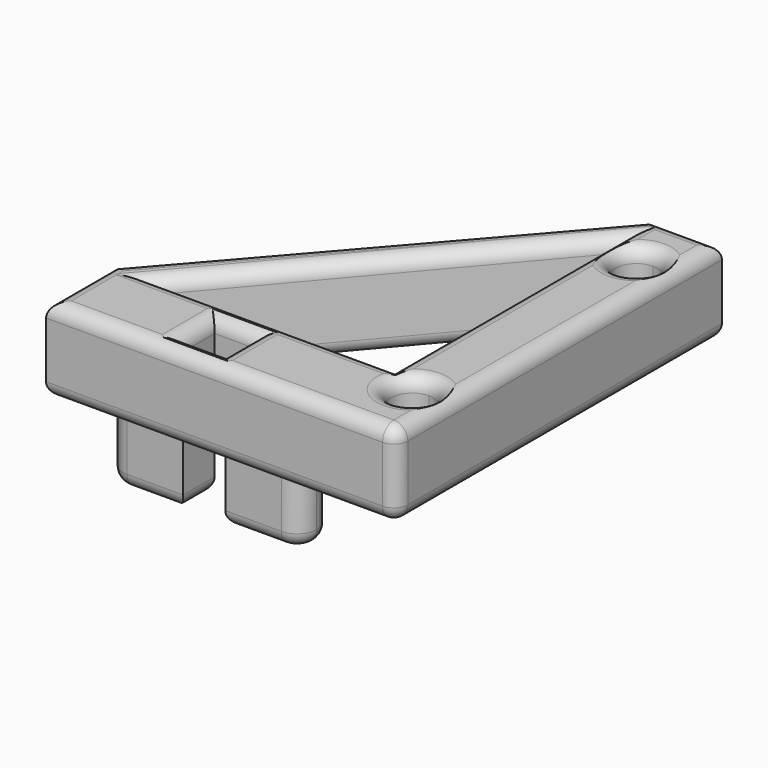
from build123d import *

# Parameters (mm, degrees)
F1_DEPTH      = 6
F2_DEPTH      = 6
F3_T1_DEPTH   = 35.4795013083
F3_T3_DEPTH   = 11
F3_T5_DEPTH   = 30
F3_T7_DEPTH   = 34
F3_T9_DEPTH   = 10
F3_T11_DEPTH  = 3
F3_T13_DEPTH  = 2.8
F3_T18_DEPTH  = 31.2488094968
F3_T24_DEPTH  = 22.5
F3_T29_DEPTH  = 19.5
F3_T39_DEPTH  = 5.5
F3_T43_DEPTH  = 5.3
F3_T50_DEPTH  = 5.5
F3_T54_DEPTH  = 5.3
F3_T61_DEPTH  = 5.3
F3_T65_DEPTH  = 5.5
F3_T72_DEPTH  = 5.5
F3_T76_DEPTH  = 5.3
F3_T83_DEPTH  = 31.2488094968
F3_T87_DEPTH  = 19.5
F3_T94_DEPTH  = 31.2488094968
F3_T98_DEPTH  = 22.5
F3_T105_DEPTH = 25
F3_T109_DEPTH = 22
F4_T1_DEPTH   = 35.4795013083
F4_T3_DEPTH   = 11
F4_T5_DEPTH   = 26.5
F4_T7_DEPTH   = 30.5
F4_T9_DEPTH   = 10
F4_T11_DEPTH  = 3
F4_T13_DEPTH  = 2.8
F4_T15_DEPTH  = 4
F4_S19_W      = 1
F4_S19_H      = 1
F4_T20_DEPTH  = 1
F4_S25_W      = 1
F4_S25_H      = 1
F4_T26_DEPTH  = 1
F4_T32_DEPTH  = 31.2488094968
F4_T38_DEPTH  = 22.5
F4_T43_DEPTH  = 19.5
F4_T53_DEPTH  = 5.5
F4_T57_DEPTH  = 5.3
F4_T64_DEPTH  = 5.5
F4_T68_DEPTH  = 5.3
F4_T75_DEPTH  = 5.5
F4_T79_DEPTH  = 5.3
F4_T86_DEPTH  = 5.3
F4_T90_DEPTH  = 5.5
F4_T97_DEPTH  = 31.2488094968
F4_T101_DEPTH = 19.5
F4_T108_DEPTH = 22.5
F4_T112_DEPTH = 31.2488094968
F4_T119_DEPTH = 25
F4_T123_DEPTH = 22
F5_DEPTH      = 5
F6_R          = 1


# Not quite as in the source:
# - a fillet or chamfer that OpenCascade refuses, or shapes differently, is made with other operations: its cross-section is extruded or revolved along the edge and cut away or added


with BuildPart() as f1:
    # F0 (on Top) → F1 (new body)
    with BuildSketch(Plane.XY):
        Polygon((0, 29), (-20, 6), (-17, 6), (0, 26), align=None)
        with BuildLine():
            Line((0, 3), (0, 0))
            Line((0, 0), (2.5, 0))
            Line((2.5, 0), (2.5, 3))
            ThreePointArc((2.5, 3), (1, 4.5), (2.5, 6))
            Line((2.5, 6), (2.5, 23))
            ThreePointArc((2.5, 23), (1, 24.5), (2.5, 26))
            Line((2.5, 26), (2.5, 29))
            Line((2.5, 29), (0, 29))
            Line((0, 29), (0, 26))
            Line((0, 26), (0, 6))
            Line((0, 6), (0, 3))
        make_face()
        with BuildLine():
            Line((2.5, 3), (2.5, 0))
            Line((2.5, 0), (5, 0))
            Line((5, 0), (5, 15))
            Line((5, 15), (5, 29))
            Line((5, 29), (2.5, 29))
            Line((2.5, 29), (2.5, 26))
            ThreePointArc((2.5, 26), (3.5606601718, 25.5606601718), (4, 24.5))
            ThreePointArc((4, 24.5), (3.5606601718, 23.4393398282), (2.5, 23))
            Line((2.5, 23), (2.5, 6))
            ThreePointArc((2.5, 6), (3.5606601718, 5.5606601718), (4, 4.5))
            ThreePointArc((4, 4.5), (3.5606601718, 3.4393398282), (2.5, 3))
        make_face()
        with BuildLine():
            Line((-3.1, 3), (0, 3))
            Line((0, 3), (0, 6))
            Line((0, 6), (-17, 6))
            Line((-17, 6), (-20, 6))
            Line((-20, 6), (-20, 3))
            Line((-20, 3), (-16.9, 3))
            ThreePointArc((-16.9, 3), (-16.4899494937, 3.9899494937), (-15.5, 4.4))
            Line((-15.5, 4.4), (-11.5, 4.4))
            Line((-11.5, 4.4), (-10, 4.4))
            Line((-10, 4.4), (-8.5, 4.4))
            Line((-8.5, 4.4), (-4.5, 4.4))
            ThreePointArc((-4.5, 4.4), (-3.5100505063, 3.9899494937), (-3.1, 3))
        make_face()
        with BuildLine():
            Line((-20, 0), (0, 0))
            Line((0, 0), (0, 3))
            Line((0, 3), (-3.1, 3))
            ThreePointArc((-3.1, 3), (-3.5100505063, 2.0100505063), (-4.5, 1.6))
            Line((-4.5, 1.6), (-8.5, 1.6))
            Line((-8.5, 1.6), (-10, 1.6))
            Line((-10, 1.6), (-11.5, 1.6))
            Line((-11.5, 1.6), (-15.5, 1.6))
            ThreePointArc((-15.5, 1.6), (-16.4899494937, 2.0100505063), (-16.9, 3))
            Line((-16.9, 3), (-20, 3))
            Line((-20, 3), (-20, 0))
        make_face()
    extrude(amount=F1_DEPTH)

    # F0 (on Top) → F2 (join)
    with BuildSketch(Plane.XY):
        with BuildLine():
            Line((-14.1, 3), (-16.9, 3))
            ThreePointArc((-16.9, 3), (-16.4899494937, 2.0100505063), (-15.5, 1.6))
            ThreePointArc((-15.5, 1.6), (-14.5100505063, 2.0100505063), (-14.1, 3))
        make_face()
        with BuildLine():
            ThreePointArc((-4.5, 1.6), (-5.4899494937, 2.0100505063), (-5.9, 3))
            Line((-5.9, 3), (-8.5, 3))
            Line((-8.5, 3), (-8.5, 1.6))
            Line((-8.5, 1.6), (-4.5, 1.6))
        make_face()
        with BuildLine():
            Line((-11.5, 3), (-14.1, 3))
            ThreePointArc((-14.1, 3), (-14.5100505063, 2.0100505063), (-15.5, 1.6))
            Line((-15.5, 1.6), (-11.5, 1.6))
            Line((-11.5, 1.6), (-11.5, 3))
        make_face()
        with BuildLine():
            ThreePointArc((-15.5, 4.4), (-14.5100505063, 3.9899494937), (-14.1, 3))
            Line((-14.1, 3), (-11.5, 3))
            Line((-11.5, 3), (-11.5, 4.4))
            Line((-11.5, 4.4), (-15.5, 4.4))
        make_face()
        with BuildLine():
            Line((-8.5, 3), (-5.9, 3))
            ThreePointArc((-5.9, 3), (-5.4899494937, 3.9899494937), (-4.5, 4.4))
            Line((-4.5, 4.4), (-8.5, 4.4))
            Line((-8.5, 4.4), (-8.5, 3))
        make_face()
        with BuildLine():
            Line((-5.9, 3), (-3.1, 3))
            ThreePointArc((-3.1, 3), (-3.5100505063, 3.9899494937), (-4.5, 4.4))
            ThreePointArc((-4.5, 4.4), (-5.4899494937, 3.9899494937), (-5.9, 3))
        make_face()
        with BuildLine():
            ThreePointArc((-4.5, 1.6), (-3.5100505063, 2.0100505063), (-3.1, 3))
            Line((-3.1, 3), (-5.9, 3))
            ThreePointArc((-5.9, 3), (-5.4899494937, 2.0100505063), (-4.5, 1.6))
        make_face()
        with BuildLine():
            ThreePointArc((-15.5, 4.4), (-16.4899494937, 3.9899494937), (-16.9, 3))
            Line((-16.9, 3), (-14.1, 3))
            ThreePointArc((-14.1, 3), (-14.5100505063, 3.9899494937), (-15.5, 4.4))
        make_face()
    extrude(amount=F2_DEPTH)

    # F3: fillet of radius 1 on 14 edges, made by hand

    # F3_s2 → F3_t1 (cut)
    with BuildSketch(Plane(origin=(15.9999731598, 18.3999691337, 0), x_dir=(0, 0, 1), z_dir=(-0.6561787149, -0.7546055222, 0))):
        with BuildLine():
            ThreePointArc((5, 19.0291827328), (5.7071067812, 18.736289514), (6, 18.0291827328))
            Line((6, 18.0291827328), (6, 19.0291827328))
            Line((6, 19.0291827328), (5, 19.0291827328))
        make_face()
    extrude(amount=F3_T1_DEPTH, mode=Mode.SUBTRACT)

    # F3_s4 → F3_t3 (cut)
    with BuildSketch(Plane.XZ.offset(-8.5)):
        with BuildLine():
            ThreePointArc((-20, 5), (-19.7071067812, 5.7071067812), (-19, 6))
            Line((-19, 6), (-20, 6))
            Line((-20, 6), (-20, 5))
        make_face()
    extrude(amount=F3_T3_DEPTH, mode=Mode.SUBTRACT)

    # F3_s6 → F3_t5 (cut)
    with BuildSketch(Plane.YZ.offset(-22.5)):
        with BuildLine():
            ThreePointArc((1, 6), (0.2928932188, 5.7071067812), (0, 5))
            Line((0, 5), (0, 6))
            Line((0, 6), (1, 6))
        make_face()
    extrude(amount=F3_T5_DEPTH, mode=Mode.SUBTRACT)

    # F3_s8 → F3_t7 (cut)
    with BuildSketch(Plane.XZ.offset(-31.5)):
        with BuildLine():
            ThreePointArc((4, 6), (4.7071067812, 5.7071067812), (5, 5))
            Line((5, 5), (5, 6))
            Line((5, 6), (4, 6))
        make_face()
    extrude(amount=F3_T7_DEPTH, mode=Mode.SUBTRACT)

    # F3_s10 → F3_t9 (cut)
    with BuildSketch(Plane.YZ.offset(-2.5)):
        with BuildLine():
            ThreePointArc((29, 5), (28.7071067812, 5.7071067812), (28, 6))
            Line((28, 6), (29, 6))
            Line((29, 6), (29, 5))
        make_face()
    extrude(amount=F3_T9_DEPTH, mode=Mode.SUBTRACT)

    # F3_s12 → F3_t11 (cut)
    with BuildSketch(Plane.YZ.offset(-11.5)):
        with BuildLine():
            ThreePointArc((5.4, 6), (4.6928932188, 5.7071067812), (4.4, 5))
            Line((4.4, 5), (4.4, 6))
            Line((4.4, 6), (5.4, 6))
        make_face()
        with BuildLine():
            ThreePointArc((0.6, 6), (1.3071067812, 5.7071067812), (1.6, 5))
            Line((1.6, 5), (1.6, 6))
            Line((1.6, 6), (0.6, 6))
        make_face()
    extrude(amount=F3_T11_DEPTH, mode=Mode.SUBTRACT)

    # F3_s14 → F3_t13 (cut)
    with BuildSketch(Plane.XZ.offset(-4.4)):
        with BuildLine():
            ThreePointArc((-7.5, 6), (-8.2071067812, 5.7071067812), (-8.5, 5))
            Line((-8.5, 5), (-8.5, 6))
            Line((-8.5, 6), (-7.5, 6))
        make_face()
        with BuildLine():
            ThreePointArc((-12.5, 6), (-11.7928932188, 5.7071067812), (-11.5, 5))
            Line((-11.5, 5), (-11.5, 6))
            Line((-11.5, 6), (-12.5, 6))
        make_face()
    extrude(amount=F3_T13_DEPTH, mode=Mode.SUBTRACT)


with BuildPart() as f3_tool16:
    # F3_s17 → F3_t18 (new body)
    with BuildSketch(Plane(origin=(-5.788932371, -6.8105086718, 0), x_dir=(0, 0, 1), z_dir=(0.6476484201, 0.7619393178, 0))):
        with BuildLine():
            ThreePointArc((6, -17.8388589225), (5.7071067812, -17.1317521413), (5, -16.8388589225))
            Line((5, -16.8388589225), (6, -16.8388589225))
            Line((6, -16.8388589225), (6, -17.8388589225))
        make_face()
    extrude(amount=F3_T18_DEPTH)

    split(bisect_by=Plane.XZ.offset(-6), keep=Keep.BOTTOM)

    split(bisect_by=Plane.YZ, keep=Keep.BOTTOM)


with BuildPart() as f1_1:
    add(f1.part)

    # F3_t15: cut F3_tool16
    add(f3_tool16.part, mode=Mode.SUBTRACT)


with BuildPart() as f3_tool22:
    # F3_s23 → F3_t24 (new body)
    with BuildSketch(Plane.XZ.offset(-28.5)):
        with BuildLine():
            ThreePointArc((1, 6), (0.2928932188, 5.7071067812), (0, 5))
            Line((0, 5), (0, 6))
            Line((0, 6), (1, 6))
        make_face()
    extrude(amount=F3_T24_DEPTH)

    split(bisect_by=Plane(origin=(-12.8301886792, 10.9056603774, 0), x_dir=(0, 0, 1), z_dir=(0.7619393178, -0.6476484201, 0)), keep=Keep.TOP)


with BuildPart() as f1_2:
    add(f1_1.part)

    # F3_t21: cut F3_tool22
    add(f3_tool22.part, mode=Mode.SUBTRACT)


with BuildPart() as f3_tool27:
    # F3_s28 → F3_t29 (new body)
    with BuildSketch(Plane.YZ):
        with BuildLine():
            ThreePointArc((5, 6), (5.7071067812, 5.7071067812), (6, 5))
            Line((6, 5), (6, 6))
            Line((6, 6), (5, 6))
        make_face()
    extrude(amount=-F3_T29_DEPTH)

    split(bisect_by=Plane(origin=(-12.8301886792, 10.9056603774, 0), x_dir=(0, 0, 1), z_dir=(0.7619393178, -0.6476484201, 0)), keep=Keep.TOP)


with BuildPart() as f1_3:
    add(f1_2.part)

    # F3_t26: cut F3_tool27
    add(f3_tool27.part, mode=Mode.SUBTRACT)

    # F3_s31 → F3_t32 (revolve, cut)
    with BuildSketch(Plane.YZ.offset(2.5)):
        with BuildLine():
            ThreePointArc((7, 6), (6.2928932188, 5.7071067812), (6, 5))
            Line((6, 5), (6, 6))
            Line((6, 6), (7, 6))
        make_face()
    revolve(axis=Axis((2.5, 4.5, 6), (0, 0, -1)), mode=Mode.SUBTRACT)

    # F3_s33 → F3_t34 (revolve, cut)
    with BuildSketch(Plane.YZ.offset(2.5)):
        with BuildLine():
            ThreePointArc((27, 6), (26.2928932188, 5.7071067812), (26, 5))
            Line((26, 5), (26, 6))
            Line((26, 6), (27, 6))
        make_face()
    revolve(axis=Axis((2.5, 24.5, 6), (0, 0, -1)), mode=Mode.SUBTRACT)


with BuildPart() as f3_tool37:
    # F3_s38 → F3_t39 (new body)
    with BuildSketch(Plane.YZ.offset(-14)):
        with BuildLine():
            ThreePointArc((5.4, 6), (4.6928932188, 5.7071067812), (4.4, 5))
            Line((4.4, 5), (4.4, 6))
            Line((4.4, 6), (5.4, 6))
        make_face()
    extrude(amount=F3_T39_DEPTH)

    split(bisect_by=Plane.YZ.offset(-11.5), keep=Keep.BOTTOM)


with BuildPart() as f3_tool41:
    # F3_s42 → F3_t43 (new body)
    with BuildSketch(Plane.XZ.offset(-1.6)):
        with BuildLine():
            ThreePointArc((-12.5, 6), (-11.7928932188, 5.7071067812), (-11.5, 5))
            Line((-11.5, 5), (-11.5, 6))
            Line((-11.5, 6), (-12.5, 6))
        make_face()
    extrude(amount=-F3_T43_DEPTH)

    split(bisect_by=Plane.XZ.offset(-4.4), keep=Keep.BOTTOM)


with BuildPart() as f3_tool37_1:
    add(f3_tool37.part)

    # F3_t45: intersect F3_tool41
    add(f3_tool41.part, mode=Mode.INTERSECT)


with BuildPart() as f1_4:
    add(f1_3.part)

    # F3_t35: cut F3_tool37
    add(f3_tool37_1.part, mode=Mode.SUBTRACT)


with BuildPart() as f3_tool48:
    # F3_s49 → F3_t50 (new body)
    with BuildSketch(Plane.YZ.offset(-11.5)):
        with BuildLine():
            ThreePointArc((5.4, 6), (4.6928932188, 5.7071067812), (4.4, 5))
            Line((4.4, 5), (4.4, 6))
            Line((4.4, 6), (5.4, 6))
        make_face()
    extrude(amount=F3_T50_DEPTH)

    split(bisect_by=Plane.YZ.offset(-8.5), keep=Keep.TOP)


with BuildPart() as f3_tool52:
    # F3_s53 → F3_t54 (new body)
    with BuildSketch(Plane.XZ.offset(-6.9)):
        with BuildLine():
            ThreePointArc((-7.5, 6), (-8.2071067812, 5.7071067812), (-8.5, 5))
            Line((-8.5, 5), (-8.5, 6))
            Line((-8.5, 6), (-7.5, 6))
        make_face()
    extrude(amount=F3_T54_DEPTH)

    split(bisect_by=Plane.XZ.offset(-4.4), keep=Keep.BOTTOM)


with BuildPart() as f3_tool48_1:
    add(f3_tool48.part)

    # F3_t56: intersect F3_tool52
    add(f3_tool52.part, mode=Mode.INTERSECT)


with BuildPart() as f1_5:
    add(f1_4.part)

    # F3_t46: cut F3_tool48
    add(f3_tool48_1.part, mode=Mode.SUBTRACT)


with BuildPart() as f3_tool59:
    # F3_s60 → F3_t61 (new body)
    with BuildSketch(Plane.XZ.offset(-4.4)):
        with BuildLine():
            ThreePointArc((-7.5, 6), (-8.2071067812, 5.7071067812), (-8.5, 5))
            Line((-8.5, 5), (-8.5, 6))
            Line((-8.5, 6), (-7.5, 6))
        make_face()
    extrude(amount=F3_T61_DEPTH)

    split(bisect_by=Plane.XZ.offset(-1.6), keep=Keep.TOP)


with BuildPart() as f3_tool63:
    # F3_s64 → F3_t65 (new body)
    with BuildSketch(Plane.YZ.offset(-6)):
        with BuildLine():
            ThreePointArc((0.6, 6), (1.3071067812, 5.7071067812), (1.6, 5))
            Line((1.6, 5), (1.6, 6))
            Line((1.6, 6), (0.6, 6))
        make_face()
    extrude(amount=-F3_T65_DEPTH)

    split(bisect_by=Plane.YZ.offset(-8.5), keep=Keep.TOP)


with BuildPart() as f3_tool59_1:
    add(f3_tool59.part)

    # F3_t67: intersect F3_tool63
    add(f3_tool63.part, mode=Mode.INTERSECT)


with BuildPart() as f1_6:
    add(f1_5.part)

    # F3_t57: cut F3_tool59
    add(f3_tool59_1.part, mode=Mode.SUBTRACT)


with BuildPart() as f3_tool70:
    # F3_s71 → F3_t72 (new body)
    with BuildSketch(Plane.YZ.offset(-8.5)):
        with BuildLine():
            ThreePointArc((0.6, 6), (1.3071067812, 5.7071067812), (1.6, 5))
            Line((1.6, 5), (1.6, 6))
            Line((1.6, 6), (0.6, 6))
        make_face()
    extrude(amount=-F3_T72_DEPTH)

    split(bisect_by=Plane.YZ.offset(-11.5), keep=Keep.BOTTOM)


with BuildPart() as f3_tool74:
    # F3_s75 → F3_t76 (new body)
    with BuildSketch(Plane.XZ.offset(0.9)):
        with BuildLine():
            ThreePointArc((-12.5, 6), (-11.7928932188, 5.7071067812), (-11.5, 5))
            Line((-11.5, 5), (-11.5, 6))
            Line((-11.5, 6), (-12.5, 6))
        make_face()
    extrude(amount=-F3_T76_DEPTH)

    split(bisect_by=Plane.XZ.offset(-1.6), keep=Keep.TOP)


with BuildPart() as f3_tool70_1:
    add(f3_tool70.part)

    # F3_t78: intersect F3_tool74
    add(f3_tool74.part, mode=Mode.INTERSECT)


with BuildPart() as f1_7:
    add(f1_6.part)

    # F3_t68: cut F3_tool70
    add(f3_tool70_1.part, mode=Mode.SUBTRACT)


with BuildPart() as f3_tool81:
    # F3_s82 → F3_t83 (new body)
    with BuildSketch(Plane(origin=(-5.788932371, -6.8105086718, 0), x_dir=(0, 0, 1), z_dir=(0.6476484201, 0.7619393178, 0))):
        with BuildLine():
            ThreePointArc((6, -17.8388589225), (5.7071067812, -17.1317521413), (5, -16.8388589225))
            Line((5, -16.8388589225), (6, -16.8388589225))
            Line((6, -16.8388589225), (6, -17.8388589225))
        make_face()
    extrude(amount=F3_T83_DEPTH)

    split(bisect_by=Plane.XZ.offset(-6), keep=Keep.TOP)


with BuildPart() as f3_tool85:
    # F3_s86 → F3_t87 (new body)
    with BuildSketch(Plane.YZ):
        with BuildLine():
            ThreePointArc((5, 6), (5.7071067812, 5.7071067812), (6, 5))
            Line((6, 5), (6, 6))
            Line((6, 6), (5, 6))
        make_face()
    extrude(amount=-F3_T87_DEPTH)

    split(bisect_by=Plane(origin=(-12.8301886792, 10.9056603774, 0), x_dir=(0, 0, 1), z_dir=(-0.7619393178, 0.6476484201, 0)), keep=Keep.TOP)


with BuildPart() as f3_tool81_1:
    add(f3_tool81.part)

    # F3_t89: intersect F3_tool85
    add(f3_tool85.part, mode=Mode.INTERSECT)


with BuildPart() as f1_8:
    add(f1_7.part)

    # F3_t79: cut F3_tool81
    add(f3_tool81_1.part, mode=Mode.SUBTRACT)


with BuildPart() as f3_tool92:
    # F3_s93 → F3_t94 (new body)
    with BuildSketch(Plane(origin=(-5.788932371, -6.8105086718, 0), x_dir=(0, 0, 1), z_dir=(0.6476484201, 0.7619393178, 0))):
        with BuildLine():
            ThreePointArc((6, -17.8388589225), (5.7071067812, -17.1317521413), (5, -16.8388589225))
            Line((5, -16.8388589225), (6, -16.8388589225))
            Line((6, -16.8388589225), (6, -17.8388589225))
        make_face()
    extrude(amount=F3_T94_DEPTH)

    split(bisect_by=Plane.YZ, keep=Keep.TOP)


with BuildPart() as f3_tool96:
    # F3_s97 → F3_t98 (new body)
    with BuildSketch(Plane.XZ.offset(-28.5)):
        with BuildLine():
            ThreePointArc((1, 6), (0.2928932188, 5.7071067812), (0, 5))
            Line((0, 5), (0, 6))
            Line((0, 6), (1, 6))
        make_face()
    extrude(amount=F3_T98_DEPTH)

    split(bisect_by=Plane(origin=(-12.8301886792, 10.9056603774, 0), x_dir=(0, 0, 1), z_dir=(-0.7619393178, 0.6476484201, 0)), keep=Keep.TOP)


with BuildPart() as f3_tool92_1:
    add(f3_tool92.part)

    # F3_t100: intersect F3_tool96
    add(f3_tool96.part, mode=Mode.INTERSECT)


with BuildPart() as f1_9:
    add(f1_8.part)

    # F3_t90: cut F3_tool92
    add(f3_tool92_1.part, mode=Mode.SUBTRACT)


with BuildPart() as f3_tool103:
    # F3_s104 → F3_t105 (new body)
    with BuildSketch(Plane.XZ.offset(-28.5)):
        with BuildLine():
            ThreePointArc((1, 6), (0.2928932188, 5.7071067812), (0, 5))
            Line((0, 5), (0, 6))
            Line((0, 6), (1, 6))
        make_face()
    extrude(amount=F3_T105_DEPTH)

    split(bisect_by=Plane.XZ.offset(-6), keep=Keep.TOP)


with BuildPart() as f3_tool107:
    # F3_s108 → F3_t109 (new body)
    with BuildSketch(Plane.YZ.offset(2.5)):
        with BuildLine():
            ThreePointArc((5, 6), (5.7071067812, 5.7071067812), (6, 5))
            Line((6, 5), (6, 6))
            Line((6, 6), (5, 6))
        make_face()
    extrude(amount=-F3_T109_DEPTH)

    split(bisect_by=Plane.YZ, keep=Keep.TOP)


with BuildPart() as f3_tool103_1:
    add(f3_tool103.part)

    # F3_t111: intersect F3_tool107
    add(f3_tool107.part, mode=Mode.INTERSECT)


with BuildPart() as f1_10:
    add(f1_9.part)

    # F3_t101: cut F3_tool103
    add(f3_tool103_1.part, mode=Mode.SUBTRACT)

    # F4: fillet of radius 1 on 15 edges, made by hand

    # F4_s2 → F4_t1 (cut)
    with BuildSketch(Plane(origin=(15.9999731598, 18.3999691337, 0), x_dir=(0, 0, 1), z_dir=(-0.6561787149, -0.7546055222, 0))):
        with BuildLine():
            ThreePointArc((1, 19.0291827328), (0.2928932188, 18.736289514), (0, 18.0291827328))
            Line((0, 18.0291827328), (0, 19.0291827328))
            Line((0, 19.0291827328), (1, 19.0291827328))
        make_face()
    extrude(amount=F4_T1_DEPTH, mode=Mode.SUBTRACT)

    # F4_s4 → F4_t3 (cut)
    with BuildSketch(Plane.XZ.offset(-8.5)):
        with BuildLine():
            ThreePointArc((-20, 1), (-19.7071067812, 0.2928932188), (-19, 0))
            Line((-19, 0), (-20, 0))
            Line((-20, 0), (-20, 1))
        make_face()
    extrude(amount=F4_T3_DEPTH, mode=Mode.SUBTRACT)

    # F4_s6 → F4_t5 (cut)
    with BuildSketch(Plane.YZ.offset(-22.5)):
        with BuildLine():
            ThreePointArc((0, 1), (0.2928932188, 0.2928932188), (1, 0))
            Line((1, 0), (0, 0))
            Line((0, 0), (0, 1))
        make_face()
    extrude(amount=F4_T5_DEPTH, mode=Mode.SUBTRACT)

    # F4_s8 → F4_t7 (cut)
    with BuildSketch(Plane.XZ.offset(-31.5)):
        with BuildLine():
            ThreePointArc((5, 1), (4.7071067812, 0.2928932188), (4, 0))
            Line((4, 0), (5, 0))
            Line((5, 0), (5, 1))
        make_face()
    extrude(amount=F4_T7_DEPTH, mode=Mode.SUBTRACT)

    # F4_s10 → F4_t9 (cut)
    with BuildSketch(Plane.YZ.offset(-2.5)):
        with BuildLine():
            ThreePointArc((29, 1), (28.7071067812, 0.2928932188), (28, 0))
            Line((28, 0), (29, 0))
            Line((29, 0), (29, 1))
        make_face()
    extrude(amount=F4_T9_DEPTH, mode=Mode.SUBTRACT)

    # F4_s12 → F4_t11 (cut)
    with BuildSketch(Plane.YZ.offset(-11.5)):
        with BuildLine():
            ThreePointArc((4.4, 1), (4.6928932188, 0.2928932188), (5.4, 0))
            Line((5.4, 0), (4.4, 0))
            Line((4.4, 0), (4.4, 1))
        make_face()
        with BuildLine():
            ThreePointArc((1.6, 1), (1.3071067812, 0.2928932188), (0.6, 0))
            Line((0.6, 0), (1.6, 0))
            Line((1.6, 0), (1.6, 1))
        make_face()
    extrude(amount=F4_T11_DEPTH, mode=Mode.SUBTRACT)

    # F4_s14 → F4_t13 (cut)
    with BuildSketch(Plane.XZ.offset(-4.4)):
        with BuildLine():
            ThreePointArc((-8.5, 1), (-8.2071067812, 0.2928932188), (-7.5, 0))
            Line((-7.5, 0), (-8.5, 0))
            Line((-8.5, 0), (-8.5, 1))
        make_face()
        with BuildLine():
            ThreePointArc((-11.5, 1), (-11.7928932188, 0.2928932188), (-12.5, 0))
            Line((-12.5, 0), (-11.5, 0))
            Line((-11.5, 0), (-11.5, 1))
        make_face()
    extrude(amount=F4_T13_DEPTH, mode=Mode.SUBTRACT)

    # F4_s16 → F4_t15 (cut)
    with BuildSketch(Plane.XY.offset(1)):
        with BuildLine():
            ThreePointArc((5, 1), (4.7071067812, 0.2928932188), (4, 0))
            Line((4, 0), (5, 0))
            Line((5, 0), (5, 1))
        make_face()
    extrude(amount=F4_T15_DEPTH, mode=Mode.SUBTRACT)


with BuildPart() as f4_tool18:
    # F4_s19 → F4_t20 (new body)
    with BuildSketch(Plane.YZ.offset(4)):
        with Locations((0.5, 5.5)):
            Rectangle(F4_S19_W, F4_S19_H)
    extrude(amount=F4_T20_DEPTH)

    # F4_s21 → F4_t22 (revolve, cut)
    with BuildSketch(Plane(origin=(4, 1, 5), x_dir=(0, 0.7071067812, -0.7071067812), z_dir=(0, -0.7071067812, -0.7071067812))):
        with BuildLine():
            ThreePointArc((0, -1), (1, 0), (0, 1))
            Line((0, 1), (0, -1))
        make_face()
    revolve(axis=Axis((4, 1, 5), (1, 0, 0)), mode=Mode.SUBTRACT)


with BuildPart() as f1_11:
    add(f1_10.part)

    # F4_t17: cut F4_tool18
    add(f4_tool18.part, mode=Mode.SUBTRACT)


with BuildPart() as f4_tool24:
    # F4_s25 → F4_t26 (new body)
    with BuildSketch(Plane.XY.offset(1)):
        with Locations((4.5, 0.5)):
            Rectangle(F4_S25_W, F4_S25_H)
    extrude(amount=-F4_T26_DEPTH)

    # F4_s27 → F4_t28 (revolve, cut)
    with BuildSketch(Plane(origin=(4, 1, 1), x_dir=(-0.7071067812, 0.7071067812, 0), z_dir=(-0.7071067812, -0.7071067812, 0))):
        with BuildLine():
            ThreePointArc((0, -1), (1, 0), (0, 1))
            Line((0, 1), (0, -1))
        make_face()
    revolve(axis=Axis((4, 1, 1), (0, 0, -1)), mode=Mode.SUBTRACT)


with BuildPart() as f1_12:
    add(f1_11.part)

    # F4_t23: cut F4_tool24
    add(f4_tool24.part, mode=Mode.SUBTRACT)


with BuildPart() as f4_tool30:
    # F4_s31 → F4_t32 (new body)
    with BuildSketch(Plane(origin=(-5.788932371, -6.8105086718, 0), x_dir=(0, 0, 1), z_dir=(0.6476484201, 0.7619393178, 0))):
        with BuildLine():
            ThreePointArc((1, -16.8388589225), (0.2928932188, -17.1317521413), (0, -17.8388589225))
            Line((0, -17.8388589225), (0, -16.8388589225))
            Line((0, -16.8388589225), (1, -16.8388589225))
        make_face()
    extrude(amount=F4_T32_DEPTH)

    split(bisect_by=Plane.YZ, keep=Keep.BOTTOM)

    split(bisect_by=Plane.XZ.offset(-6), keep=Keep.BOTTOM)


with BuildPart() as f1_13:
    add(f1_12.part)

    # F4_t29: cut F4_tool30
    add(f4_tool30.part, mode=Mode.SUBTRACT)


with BuildPart() as f4_tool36:
    # F4_s37 → F4_t38 (new body)
    with BuildSketch(Plane.XZ.offset(-28.5)):
        with BuildLine():
            ThreePointArc((0, 1), (0.2928932188, 0.2928932188), (1, 0))
            Line((1, 0), (0, 0))
            Line((0, 0), (0, 1))
        make_face()
    extrude(amount=F4_T38_DEPTH)

    split(bisect_by=Plane(origin=(-12.8301886792, 10.9056603774, 0), x_dir=(0, 0, 1), z_dir=(0.7619393178, -0.6476484201, 0)), keep=Keep.TOP)


with BuildPart() as f1_14:
    add(f1_13.part)

    # F4_t35: cut F4_tool36
    add(f4_tool36.part, mode=Mode.SUBTRACT)


with BuildPart() as f4_tool41:
    # F4_s42 → F4_t43 (new body)
    with BuildSketch(Plane.YZ):
        with BuildLine():
            ThreePointArc((6, 1), (5.7071067812, 0.2928932188), (5, 0))
            Line((5, 0), (6, 0))
            Line((6, 0), (6, 1))
        make_face()
    extrude(amount=-F4_T43_DEPTH)

    split(bisect_by=Plane(origin=(-12.8301886792, 10.9056603774, 0), x_dir=(0, 0, 1), z_dir=(0.7619393178, -0.6476484201, 0)), keep=Keep.TOP)


with BuildPart() as f1_15:
    add(f1_14.part)

    # F4_t40: cut F4_tool41
    add(f4_tool41.part, mode=Mode.SUBTRACT)

    # F4_s45 → F4_t46 (revolve, cut)
    with BuildSketch(Plane.YZ.offset(2.5)):
        with BuildLine():
            ThreePointArc((6, 1), (6.2928932188, 0.2928932188), (7, 0))
            Line((7, 0), (6, 0))
            Line((6, 0), (6, 1))
        make_face()
    revolve(axis=Axis((2.5, 4.5, 0), (0, 0, -1)), mode=Mode.SUBTRACT)

    # F4_s47 → F4_t48 (revolve, cut)
    with BuildSketch(Plane.YZ.offset(2.5)):
        with BuildLine():
            ThreePointArc((26, 1), (26.2928932188, 0.2928932188), (27, 0))
            Line((27, 0), (26, 0))
            Line((26, 0), (26, 1))
        make_face()
    revolve(axis=Axis((2.5, 24.5, 0), (0, 0, -1)), mode=Mode.SUBTRACT)


with BuildPart() as f4_tool51:
    # F4_s52 → F4_t53 (new body)
    with BuildSketch(Plane.YZ.offset(-14)):
        with BuildLine():
            ThreePointArc((4.4, 1), (4.6928932188, 0.2928932188), (5.4, 0))
            Line((5.4, 0), (4.4, 0))
            Line((4.4, 0), (4.4, 1))
        make_face()
    extrude(amount=F4_T53_DEPTH)

    split(bisect_by=Plane.YZ.offset(-11.5), keep=Keep.BOTTOM)


with BuildPart() as f4_tool55:
    # F4_s56 → F4_t57 (new body)
    with BuildSketch(Plane.XZ.offset(-1.6)):
        with BuildLine():
            ThreePointArc((-11.5, 1), (-11.7928932188, 0.2928932188), (-12.5, 0))
            Line((-12.5, 0), (-11.5, 0))
            Line((-11.5, 0), (-11.5, 1))
        make_face()
    extrude(amount=-F4_T57_DEPTH)

    split(bisect_by=Plane.XZ.offset(-4.4), keep=Keep.BOTTOM)


with BuildPart() as f4_tool51_1:
    add(f4_tool51.part)

    # F4_t59: intersect F4_tool55
    add(f4_tool55.part, mode=Mode.INTERSECT)


with BuildPart() as f1_16:
    add(f1_15.part)

    # F4_t49: cut F4_tool51
    add(f4_tool51_1.part, mode=Mode.SUBTRACT)


with BuildPart() as f4_tool62:
    # F4_s63 → F4_t64 (new body)
    with BuildSketch(Plane.YZ.offset(-11.5)):
        with BuildLine():
            ThreePointArc((4.4, 1), (4.6928932188, 0.2928932188), (5.4, 0))
            Line((5.4, 0), (4.4, 0))
            Line((4.4, 0), (4.4, 1))
        make_face()
    extrude(amount=F4_T64_DEPTH)

    split(bisect_by=Plane.YZ.offset(-8.5), keep=Keep.TOP)


with BuildPart() as f4_tool66:
    # F4_s67 → F4_t68 (new body)
    with BuildSketch(Plane.XZ.offset(-6.9)):
        with BuildLine():
            ThreePointArc((-8.5, 1), (-8.2071067812, 0.2928932188), (-7.5, 0))
            Line((-7.5, 0), (-8.5, 0))
            Line((-8.5, 0), (-8.5, 1))
        make_face()
    extrude(amount=F4_T68_DEPTH)

    split(bisect_by=Plane.XZ.offset(-4.4), keep=Keep.BOTTOM)


with BuildPart() as f4_tool62_1:
    add(f4_tool62.part)

    # F4_t70: intersect F4_tool66
    add(f4_tool66.part, mode=Mode.INTERSECT)


with BuildPart() as f1_17:
    add(f1_16.part)

    # F4_t60: cut F4_tool62
    add(f4_tool62_1.part, mode=Mode.SUBTRACT)


with BuildPart() as f4_tool73:
    # F4_s74 → F4_t75 (new body)
    with BuildSketch(Plane.YZ.offset(-6)):
        with BuildLine():
            ThreePointArc((1.6, 1), (1.3071067812, 0.2928932188), (0.6, 0))
            Line((0.6, 0), (1.6, 0))
            Line((1.6, 0), (1.6, 1))
        make_face()
    extrude(amount=-F4_T75_DEPTH)

    split(bisect_by=Plane.YZ.offset(-8.5), keep=Keep.TOP)


with BuildPart() as f4_tool77:
    # F4_s78 → F4_t79 (new body)
    with BuildSketch(Plane.XZ.offset(-4.4)):
        with BuildLine():
            ThreePointArc((-8.5, 1), (-8.2071067812, 0.2928932188), (-7.5, 0))
            Line((-7.5, 0), (-8.5, 0))
            Line((-8.5, 0), (-8.5, 1))
        make_face()
    extrude(amount=F4_T79_DEPTH)

    split(bisect_by=Plane.XZ.offset(-1.6), keep=Keep.TOP)


with BuildPart() as f4_tool73_1:
    add(f4_tool73.part)

    # F4_t81: intersect F4_tool77
    add(f4_tool77.part, mode=Mode.INTERSECT)


with BuildPart() as f1_18:
    add(f1_17.part)

    # F4_t71: cut F4_tool73
    add(f4_tool73_1.part, mode=Mode.SUBTRACT)


with BuildPart() as f4_tool84:
    # F4_s85 → F4_t86 (new body)
    with BuildSketch(Plane.XZ.offset(0.9)):
        with BuildLine():
            ThreePointArc((-11.5, 1), (-11.7928932188, 0.2928932188), (-12.5, 0))
            Line((-12.5, 0), (-11.5, 0))
            Line((-11.5, 0), (-11.5, 1))
        make_face()
    extrude(amount=-F4_T86_DEPTH)

    split(bisect_by=Plane.XZ.offset(-1.6), keep=Keep.TOP)


with BuildPart() as f4_tool88:
    # F4_s89 → F4_t90 (new body)
    with BuildSketch(Plane.YZ.offset(-8.5)):
        with BuildLine():
            ThreePointArc((1.6, 1), (1.3071067812, 0.2928932188), (0.6, 0))
            Line((0.6, 0), (1.6, 0))
            Line((1.6, 0), (1.6, 1))
        make_face()
    extrude(amount=-F4_T90_DEPTH)

    split(bisect_by=Plane.YZ.offset(-11.5), keep=Keep.BOTTOM)


with BuildPart() as f4_tool84_1:
    add(f4_tool84.part)

    # F4_t92: intersect F4_tool88
    add(f4_tool88.part, mode=Mode.INTERSECT)


with BuildPart() as f1_19:
    add(f1_18.part)

    # F4_t82: cut F4_tool84
    add(f4_tool84_1.part, mode=Mode.SUBTRACT)


with BuildPart() as f4_tool95:
    # F4_s96 → F4_t97 (new body)
    with BuildSketch(Plane(origin=(-5.788932371, -6.8105086718, 0), x_dir=(0, 0, 1), z_dir=(0.6476484201, 0.7619393178, 0))):
        with BuildLine():
            ThreePointArc((1, -16.8388589225), (0.2928932188, -17.1317521413), (0, -17.8388589225))
            Line((0, -17.8388589225), (0, -16.8388589225))
            Line((0, -16.8388589225), (1, -16.8388589225))
        make_face()
    extrude(amount=F4_T97_DEPTH)

    split(bisect_by=Plane.XZ.offset(-6), keep=Keep.TOP)


with BuildPart() as f4_tool99:
    # F4_s100 → F4_t101 (new body)
    with BuildSketch(Plane.YZ):
        with BuildLine():
            ThreePointArc((6, 1), (5.7071067812, 0.2928932188), (5, 0))
            Line((5, 0), (6, 0))
            Line((6, 0), (6, 1))
        make_face()
    extrude(amount=-F4_T101_DEPTH)

    split(bisect_by=Plane(origin=(-12.8301886792, 10.9056603774, 0), x_dir=(0, 0, 1), z_dir=(-0.7619393178, 0.6476484201, 0)), keep=Keep.TOP)


with BuildPart() as f4_tool95_1:
    add(f4_tool95.part)

    # F4_t103: intersect F4_tool99
    add(f4_tool99.part, mode=Mode.INTERSECT)


with BuildPart() as f1_20:
    add(f1_19.part)

    # F4_t93: cut F4_tool95
    add(f4_tool95_1.part, mode=Mode.SUBTRACT)


with BuildPart() as f4_tool106:
    # F4_s107 → F4_t108 (new body)
    with BuildSketch(Plane.XZ.offset(-28.5)):
        with BuildLine():
            ThreePointArc((0, 1), (0.2928932188, 0.2928932188), (1, 0))
            Line((1, 0), (0, 0))
            Line((0, 0), (0, 1))
        make_face()
    extrude(amount=F4_T108_DEPTH)

    split(bisect_by=Plane(origin=(-12.8301886792, 10.9056603774, 0), x_dir=(0, 0, 1), z_dir=(-0.7619393178, 0.6476484201, 0)), keep=Keep.TOP)


with BuildPart() as f4_tool110:
    # F4_s111 → F4_t112 (new body)
    with BuildSketch(Plane(origin=(-5.788932371, -6.8105086718, 0), x_dir=(0, 0, 1), z_dir=(0.6476484201, 0.7619393178, 0))):
        with BuildLine():
            ThreePointArc((1, -16.8388589225), (0.2928932188, -17.1317521413), (0, -17.8388589225))
            Line((0, -17.8388589225), (0, -16.8388589225))
            Line((0, -16.8388589225), (1, -16.8388589225))
        make_face()
    extrude(amount=F4_T112_DEPTH)

    split(bisect_by=Plane.YZ, keep=Keep.TOP)


with BuildPart() as f4_tool106_1:
    add(f4_tool106.part)

    # F4_t114: intersect F4_tool110
    add(f4_tool110.part, mode=Mode.INTERSECT)


with BuildPart() as f1_21:
    add(f1_20.part)

    # F4_t104: cut F4_tool106
    add(f4_tool106_1.part, mode=Mode.SUBTRACT)


with BuildPart() as f4_tool117:
    # F4_s118 → F4_t119 (new body)
    with BuildSketch(Plane.XZ.offset(-28.5)):
        with BuildLine():
            ThreePointArc((0, 1), (0.2928932188, 0.2928932188), (1, 0))
            Line((1, 0), (0, 0))
            Line((0, 0), (0, 1))
        make_face()
    extrude(amount=F4_T119_DEPTH)

    split(bisect_by=Plane.XZ.offset(-6), keep=Keep.TOP)


with BuildPart() as f4_tool121:
    # F4_s122 → F4_t123 (new body)
    with BuildSketch(Plane.YZ.offset(2.5)):
        with BuildLine():
            ThreePointArc((6, 1), (5.7071067812, 0.2928932188), (5, 0))
            Line((5, 0), (6, 0))
            Line((6, 0), (6, 1))
        make_face()
    extrude(amount=-F4_T123_DEPTH)

    split(bisect_by=Plane.YZ, keep=Keep.TOP)


with BuildPart() as f4_tool117_1:
    add(f4_tool117.part)

    # F4_t125: intersect F4_tool121
    add(f4_tool121.part, mode=Mode.INTERSECT)


with BuildPart() as f1_22:
    add(f1_21.part)

    # F4_t115: cut F4_tool117
    add(f4_tool117_1.part, mode=Mode.SUBTRACT)

    # F0 (on Top) → F5 (join)
    with BuildSketch(Plane.XY):
        with BuildLine():
            Line((-14.1, 3), (-16.9, 3))
            ThreePointArc((-16.9, 3), (-16.4899494937, 2.0100505063), (-15.5, 1.6))
            ThreePointArc((-15.5, 1.6), (-14.5100505063, 2.0100505063), (-14.1, 3))
        make_face()
        with BuildLine():
            ThreePointArc((-15.5, 4.4), (-16.4899494937, 3.9899494937), (-16.9, 3))
            Line((-16.9, 3), (-14.1, 3))
            ThreePointArc((-14.1, 3), (-14.5100505063, 3.9899494937), (-15.5, 4.4))
        make_face()
        with BuildLine():
            ThreePointArc((-15.5, 4.4), (-14.5100505063, 3.9899494937), (-14.1, 3))
            Line((-14.1, 3), (-11.5, 3))
            Line((-11.5, 3), (-11.5, 4.4))
            Line((-11.5, 4.4), (-15.5, 4.4))
        make_face()
        with BuildLine():
            Line((-8.5, 3), (-5.9, 3))
            ThreePointArc((-5.9, 3), (-5.4899494937, 3.9899494937), (-4.5, 4.4))
            Line((-4.5, 4.4), (-8.5, 4.4))
            Line((-8.5, 4.4), (-8.5, 3))
        make_face()
        with BuildLine():
            ThreePointArc((-4.5, 1.6), (-5.4899494937, 2.0100505063), (-5.9, 3))
            Line((-5.9, 3), (-8.5, 3))
            Line((-8.5, 3), (-8.5, 1.6))
            Line((-8.5, 1.6), (-4.5, 1.6))
        make_face()
        with BuildLine():
            Line((-11.5, 3), (-14.1, 3))
            ThreePointArc((-14.1, 3), (-14.5100505063, 2.0100505063), (-15.5, 1.6))
            Line((-15.5, 1.6), (-11.5, 1.6))
            Line((-11.5, 1.6), (-11.5, 3))
        make_face()
        with BuildLine():
            ThreePointArc((-4.5, 1.6), (-3.5100505063, 2.0100505063), (-3.1, 3))
            Line((-3.1, 3), (-5.9, 3))
            ThreePointArc((-5.9, 3), (-5.4899494937, 2.0100505063), (-4.5, 1.6))
        make_face()
        with BuildLine():
            Line((-5.9, 3), (-3.1, 3))
            ThreePointArc((-3.1, 3), (-3.5100505063, 3.9899494937), (-4.5, 4.4))
            ThreePointArc((-4.5, 4.4), (-5.4899494937, 3.9899494937), (-5.9, 3))
        make_face()
    extrude(amount=-F5_DEPTH)

    # F6
    f6_edges = [f1_22.edges().sort_by_distance(p)[0] for p in [
        (-6.5, 4.4, -5),
        (-8.5, 3, -5),
        (-6.5, 1.6, -5),
        (-3.1, 3, -5),
        (-13.5, 4.4, -5),
        (-16.9, 3, -5),
        (-13.5, 1.6, -5),
        (-11.5, 3, -5),
    ]]
    fillet(f6_edges, radius=F6_R)


solid = f1_22.part
